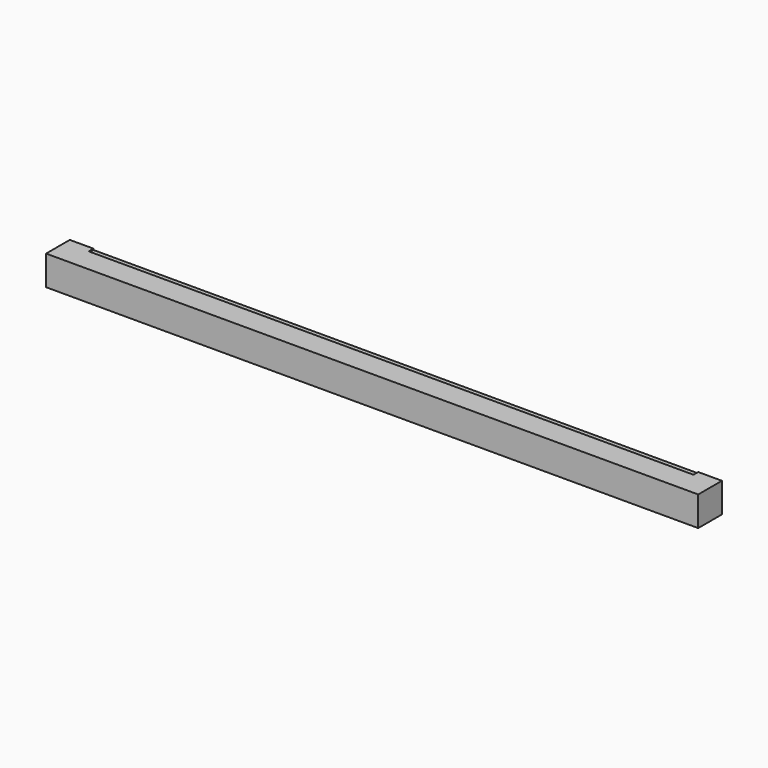
from build123d import *

# Parameters (mm, degrees)
F0_W      = 1100
F0_H      = 50
F1_DEPTH  = 50
F2_W      = 30
F2_H      = 30
F3_DEPTH  = 40
F5_W      = 1020
F5_H      = 10
F6_DEPTH  = 2
F7_W      = 1030
F7_H      = 2
F8_DEPTH  = 5
F9_W      = 30
F9_H      = 30
F10_DEPTH = 40
F11_W     = 20
F11_H     = 4
F12_DEPTH = 30


# Not quite as in the source:
# - a pattern or mirror of a feature is missing from the dataset's text; its kind, count and spacing are read off the source's solid


with BuildPart() as f1:
    # F0 (on Top) → F1 (new body)
    with BuildSketch(Plane.XY):
        with Locations((-550, -25)):
            Rectangle(F0_W, F0_H)
    extrude(amount=F1_DEPTH)

    # F2 (on face) → F3 (cut)
    with BuildSketch(Plane(origin=(0, 0, 0), x_dir=(1, 0, 0), z_dir=(0, 0, -1))):
        with Locations((-25, 25)):
            Rectangle(F2_W, F2_H)
    f3 = extrude(amount=-F3_DEPTH, mode=Mode.SUBTRACT)

    # F3_copies: F3 across plane
    add(f3.mirror(Plane(origin=(-550, 0, 0), x_dir=(0, 0, -1), z_dir=(-1, 0, 0))), mode=Mode.SUBTRACT)

    # F5 (on face) → F6 (cut)
    with BuildSketch(Plane.XY.offset(50)):
        with Locations((-550, -5)):
            Rectangle(F5_W, F5_H)
    extrude(amount=-F6_DEPTH, mode=Mode.SUBTRACT)

    # F7 (on face) → F8 (cut)
    with BuildSketch(Plane(origin=(0, 0, 0), x_dir=(-1, 0, 0), z_dir=(0, 1, 0))):
        with Locations((550, 46)):
            Rectangle(F7_W, F7_H)
    extrude(amount=-F8_DEPTH, mode=Mode.SUBTRACT)

    # F9 (on face) → F10 (cut)
    with BuildSketch(Plane(origin=(0, 0, 0), x_dir=(-1, 0, 0), z_dir=(0, 1, 0))):
        with Locations((25, 25)):
            Rectangle(F9_W, F9_H)
    f10 = extrude(amount=-F10_DEPTH, mode=Mode.SUBTRACT)

    # F10_copies: F10 across plane
    add(f10.mirror(Plane(origin=(-550, 0, 0), x_dir=(0, 0, -1), z_dir=(-1, 0, 0))), mode=Mode.SUBTRACT)

    # F11 (on face) → F12 (cut)
    with BuildSketch(Plane(origin=(0, 0, 0), x_dir=(-1, 0, 0), z_dir=(0, 1, 0))):
        with Locations((550, 40)):
            Rectangle(F11_W, F11_H)
    extrude(amount=-F12_DEPTH, mode=Mode.SUBTRACT)


solid = f1.part
